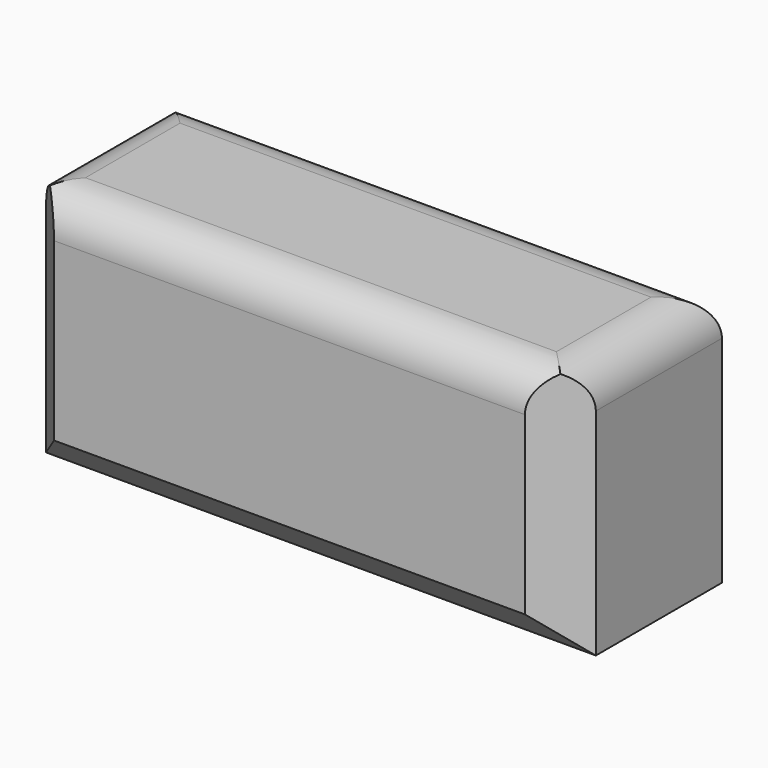
from build123d import *

# Parameters (mm, degrees)
F1_DEPTH    = 25.4
F2_R        = 5.08
F3_T1_DEPTH = 53.8847270698
F3_T3_DEPTH = 97.0179937739


# Not quite as in the source:
# - a fillet or chamfer that OpenCascade refuses, or shapes differently, is made with other operations: its cross-section is extruded or revolved along the edge and cut away or added


with BuildPart() as f1:
    # F0 (on Front) → F1 (new body)
    with BuildSketch(Plane.XZ):
        with BuildLine():
            ThreePointArc((-26.0082527554, 9.7501287237), (-33.751696872, 20.4773638636), (-46.3714562356, 16.5054406347))
            Line((-46.3714562356, 16.5054406347), (-46.3714562356, 2.9948168126))
            ThreePointArc((-46.3714562356, 2.9948168126), (-33.751696872, -0.9771064163), (-26.0082527554, 9.7501287237))
        make_face()
        with BuildLine():
            Line((24.5182383806, 25.2565909177), (-46.3714562356, 25.2565909177))
            Line((-46.3714562356, 25.2565909177), (-46.3714562356, 16.5054406347))
            ThreePointArc((-46.3714562356, 16.5054406347), (-33.751696872, 20.4773638636), (-26.0082527554, 9.7501287237))
            ThreePointArc((-26.0082527554, 9.7501287237), (-33.751696872, -0.9771064163), (-46.3714562356, 2.9948168126))
            Line((-46.3714562356, 2.9948168126), (-46.3714562356, -7.5798369944))
            Line((-46.3714562356, -7.5798369944), (24.5182383806, -7.5798369944))
            Line((24.5182383806, -7.5798369944), (24.5182383806, 25.2565909177))
        make_face()
    extrude(amount=F1_DEPTH)

    # F2
    f2_edges = [f1.edges().sort_by_distance(p)[0] for p in [
        (24.518238, -12.7, 25.256591),
        (-46.371456, -12.7, 25.256591),
        (-10.926609, 0, 25.256591),
        (-10.926609, -25.4, 25.256591),
    ]]
    fillet(f2_edges, radius=F2_R)

    # F3: chamfer of 5.08 on 4 edges, made by hand

    # F3_s2 → F3_t1 (cut)
    with BuildSketch(Plane.XY.offset(-20.6439865733)):
        Polygon((-41.2914562356, -25.4), (-46.3714562356, -20.32), (-46.3714562356, -25.4), align=None)
        Polygon((24.5182383806, -20.32), (19.4382383806, -25.4), (24.5182383806, -25.4), align=None)
    extrude(amount=F3_T1_DEPTH, mode=Mode.SUBTRACT)

    # F3_s4 → F3_t3 (cut)
    with BuildSketch(Plane.YZ.offset(-59.4356058145)):
        Polygon((-20.32, -7.5798369944), (-25.4, -2.4998369944), (-25.4, -7.5798369944), align=None)
    extrude(amount=F3_T3_DEPTH, mode=Mode.SUBTRACT)


solid = f1.part
